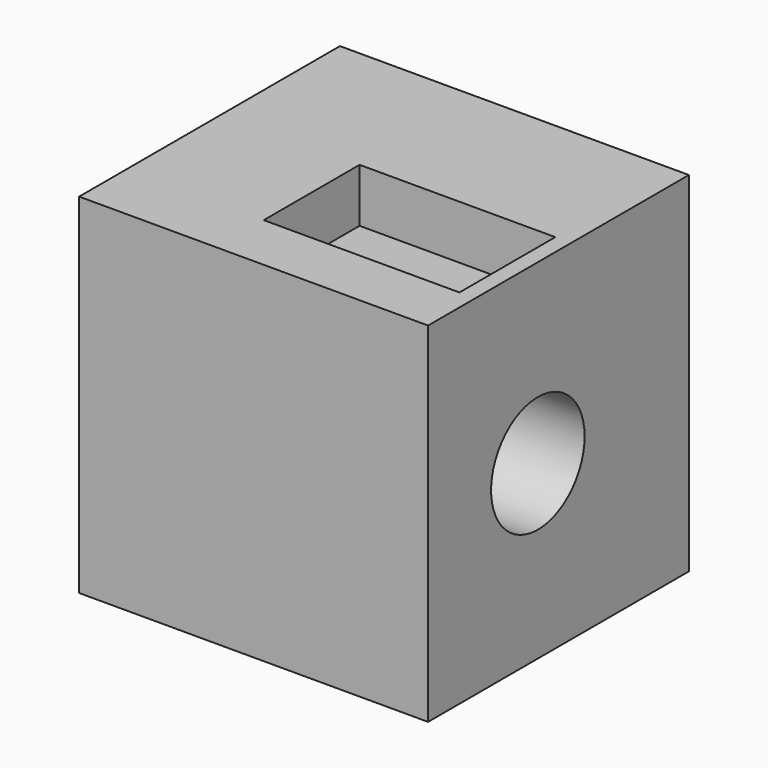
from build123d import *

# Parameters (mm, degrees)
F1_W     = 165.1
F1_H     = 154.2292288029
F2_DEPTH = 165.1
F3_R     = 27.6489440809
F4_DEPTH = 247.396
F5_W     = 92.6118567586
F5_H     = 56.6696990281
F6_DEPTH = 25.4


# Not quite as in the source:
# - a variable given as a bare number and used for a length is read in inches; the dataset says mm whatever the document's units were


with BuildPart() as f2:
    # F1 (on Top) → F2 (new body)
    with BuildSketch(Plane.XY):
        Rectangle(F1_W, F1_H)
    extrude(amount=F2_DEPTH)

    # F3 (on face) → F4 (cut)
    with BuildSketch(Plane.YZ.offset(82.55)):
        with Locations((-12.199181132, 81.3155397773)):
            Circle(F3_R)
    extrude(amount=-F4_DEPTH, mode=Mode.SUBTRACT)

    # F5 (on face) → F6 (cut)
    with BuildSketch(Plane.XY.offset(165.1)):
        with Locations((28.7659913301, -20.8643507212)):
            Rectangle(F5_W, F5_H)
    extrude(amount=-F6_DEPTH, mode=Mode.SUBTRACT)


solid = f2.part
